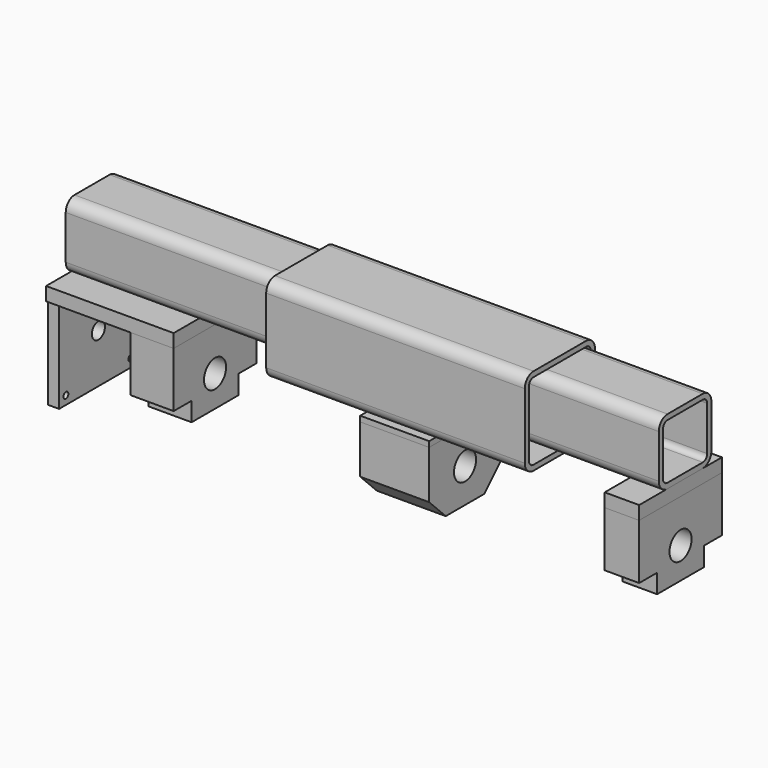
from build123d import *

# Parameters (mm, degrees)
F4_R      = 1.7859375
F4_R_2    = 4.7625
F6_DEPTH  = 6.35
F7_START  = 49
F3_R      = 8
F7_DEPTH  = 25
F8_START  = 124
F8_DEPTH  = 150
F9_DEPTH  = 344
F10_START = 179
F0_R      = 8
F10_DEPTH = 40
F3_W      = 60
F3_H      = 7.8270026548
F11_DEPTH = 74
F12_START = 324
F12_DEPTH = 20
F13_START = 324
F13_DEPTH = 20
F14_START = 179
F14_DEPTH = 40


# Not quite as in the source:
# - ends of sketch curves that miss each other by under 0.0002 mm in the source are joined


with BuildPart() as f6:
    # F4 (on Right) → F6 (new body, through all)
    with BuildSketch(Plane.YZ):
        with BuildLine():
            ThreePointArc((-22.5073684961, 24.9999973452), (-21.9607159701, 24.3647079392), (-21.7640625, 23.55))
            ThreePointArc((-21.7640625, 23.55), (-24.3647079392, 21.9607159701), (-24.5926315039, 24.9999973452))
            Line((-24.5926315039, 24.9999973452), (-28.5, 24.9999973452))
            Line((-28.5, 24.9999973452), (-28.5, -28.5))
            Line((-28.5, -28.5), (28.5, -28.5))
            Line((28.5, -28.5), (28.5, 24.9999973452))
            Line((28.5, 24.9999973452), (24.5926315039, 24.9999973452))
            ThreePointArc((24.5926315039, 24.9999973452), (25.1392840299, 24.3647079392), (25.3359375, 23.55))
            ThreePointArc((25.3359375, 23.55), (22.7352920608, 21.9607159701), (22.5073684961, 24.9999973452))
            Line((22.5073684961, 24.9999973452), (-22.5073684961, 24.9999973452))
        make_face()
        with Locations((-23.55, -23.55)):
            Circle(F4_R, mode=Mode.SUBTRACT)
        with Locations((23.55, -23.55)):
            Circle(F4_R, mode=Mode.SUBTRACT)
        Circle(F4_R_2, mode=Mode.SUBTRACT)
    extrude(amount=F6_DEPTH)


with BuildPart() as f7:
    # F3 (on Right) → F7 (new body)
    with BuildSketch(Plane.YZ.offset(F7_START)):
        Polygon((30, 24.9999973452), (-30, 25.0000026548), (-30, -6.9999973452), (-17, -6.9999973452), (-17, -17.9999973452), (17, -17.9999973452), (17, -6.9999973452), (30, -6.9999973452), align=None)
        Circle(F3_R, mode=Mode.SUBTRACT)
    extrude(amount=F7_DEPTH)


with BuildPart() as f8:
    # F1 (on Right) → F8 (new body)
    with BuildSketch(Plane.YZ.offset(F8_START)):
        with BuildLine():
            ThreePointArc((25.4, 67.625), (23.5401280605, 72.1151280605), (19.05, 73.975))
            Line((19.05, 73.975), (-19.05, 73.975))
            ThreePointArc((-19.05, 73.975), (-23.5401280605, 72.1151280605), (-25.4, 67.625))
            Line((-25.4, 67.625), (-25.4, 29.525))
            ThreePointArc((-25.4, 29.525), (-23.5401280605, 25.0348719395), (-19.05, 23.175))
            Line((-19.05, 23.175), (19.05, 23.175))
            ThreePointArc((19.05, 23.175), (23.5401280605, 25.0348719395), (25.4, 29.525))
            Line((25.4, 29.525), (25.4, 67.625))
        make_face()
        with BuildLine():
            Line((-19.177, 70.927), (19.177, 70.927))
            ThreePointArc((19.177, 70.927), (21.4220640303, 69.9970640303), (22.352, 67.752))
            Line((22.352, 67.752), (22.352, 29.398))
            ThreePointArc((22.352, 29.398), (21.4220640303, 27.1529359697), (19.177, 26.223))
            Line((19.177, 26.223), (-19.177, 26.223))
            ThreePointArc((-19.177, 26.223), (-21.4220640303, 27.1529359697), (-22.352, 29.398))
            Line((-22.352, 29.398), (-22.352, 67.752))
            ThreePointArc((-22.352, 67.752), (-21.4220640303, 69.9970640303), (-19.177, 70.927))
        make_face(mode=Mode.SUBTRACT)
    extrude(amount=F8_DEPTH)


with BuildPart() as f9:
    # F2 (on Right) → F9 (new body, through all)
    with BuildSketch(Plane.YZ):
        with BuildLine():
            ThreePointArc((22.352, 64.577), (20.4921280605, 69.0671280605), (16.002, 70.927))
            Line((16.002, 70.927), (-9.398, 70.927))
            ThreePointArc((-9.398, 70.927), (-13.8881280605, 69.0671280605), (-15.748, 64.577))
            Line((-15.748, 64.577), (-15.748, 39.177))
            ThreePointArc((-15.748, 39.177), (-13.8881280605, 34.6868719395), (-9.398, 32.827))
            Line((-9.398, 32.827), (16.002, 32.827))
            ThreePointArc((16.002, 32.827), (20.4921280605, 34.6868719395), (22.352, 39.177))
            Line((22.352, 39.177), (22.352, 64.577))
        make_face()
        with BuildLine():
            Line((-9.525, 67.879), (16.129, 67.879))
            ThreePointArc((16.129, 67.879), (18.3740640303, 66.9490640303), (19.304, 64.704))
            Line((19.304, 64.704), (19.304, 39.05))
            ThreePointArc((19.304, 39.05), (18.3740640303, 36.8049359697), (16.129, 35.875))
            Line((16.129, 35.875), (-9.525, 35.875))
            ThreePointArc((-9.525, 35.875), (-11.7700640303, 36.8049359697), (-12.7, 39.05))
            Line((-12.7, 39.05), (-12.7, 64.704))
            ThreePointArc((-12.7, 64.704), (-11.7700640303, 66.9490640303), (-9.525, 67.879))
        make_face(mode=Mode.SUBTRACT)
    extrude(amount=F9_DEPTH)


with BuildPart() as f10:
    # F0 (on Right) → F10 (new body)
    with BuildSketch(Plane.YZ.offset(F10_START)):
        Polygon((26, 20), (-26, 20), (-26, -7.9791847198), (-13.9791847198, -20), (13.9791847198, -20), (26, -7.9791847198), align=None)
        Circle(F0_R, mode=Mode.SUBTRACT)
    extrude(amount=F10_DEPTH)


with BuildPart() as f11:
    # F3 (on Right) → F11 (new body, through all)
    with BuildSketch(Plane.YZ):
        with Locations((0, 28.9134986726)):
            Rectangle(F3_W, F3_H)
    extrude(amount=F11_DEPTH)


with BuildPart() as f12:
    # F3 (on Right) → F12 (new body)
    with BuildSketch(Plane.YZ.offset(F12_START)):
        Polygon((30, 24.9999973452), (-30, 25.0000026548), (-30, -6.9999973452), (-17, -6.9999973452), (-17, -17.9999973452), (17, -17.9999973452), (17, -6.9999973452), (30, -6.9999973452), align=None)
        Circle(F3_R, mode=Mode.SUBTRACT)
    extrude(amount=F12_DEPTH)


with BuildPart() as f13:
    # F3 (on Right) → F13 (new body)
    with BuildSketch(Plane.YZ.offset(F13_START)):
        with Locations((0, 28.9134986726)):
            Rectangle(F3_W, F3_H)
    extrude(amount=F13_DEPTH)


with BuildPart() as f14:
    # F1 (on Right) → F14 (new body)
    with BuildSketch(Plane.YZ.offset(F14_START)):
        Polygon((26, 23.175), (19.05, 23.175), (-19.05, 23.175), (-26, 23.175), (-26, 20), (26, 20), align=None)
    extrude(amount=F14_DEPTH)


solid = Compound([f6.part, f7.part, f8.part, f9.part, f10.part, f11.part, f12.part, f13.part, f14.part])
